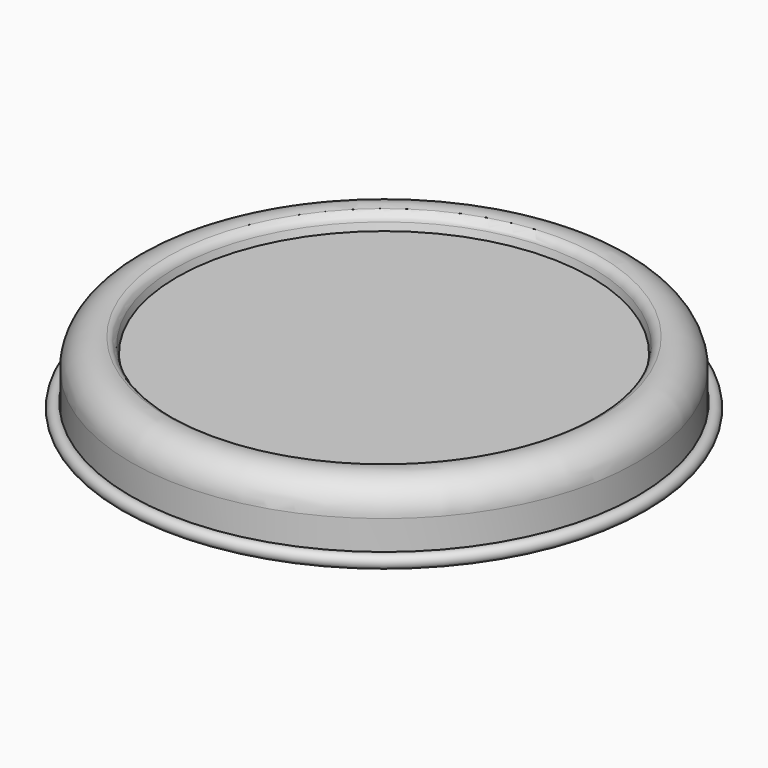
from build123d import *

# Parameters (mm, degrees)
F0_R     = 19.25
F1_DEPTH = 2.6185
F6_T     = 0.15


# Not quite as in the source:
# - a shell that OpenCascade refuses in one call is made with other operations: the cavity is built on its own and cut out


with BuildPart() as f1:
    # F0 (on Top) → F1 (new body)
    with BuildSketch(Plane.XY):
        Circle(F0_R)
    extrude(amount=F1_DEPTH)

    # F2 (on Front) → F3 (revolve)
    with BuildSketch(Plane.XZ):
        with BuildLine():
            Line((-19.39, 0.28), (-19.3, 0.4))
            ThreePointArc((-19.3, 0.4), (-20.0472135955, -0.2236067977), (-19.1, 0))
            Line((-19.1, 0), (-19.25, 0))
            ThreePointArc((-19.25, 0), (-19.9130495168, -0.1565247584), (-19.39, 0.28))
        make_face()
    revolve(axis=Axis((0, 0, 0), (0, 0, 1)))

    # F4 (on Front) → F5 (revolve)
    with BuildSketch(Plane.XZ):
        with BuildLine():
            ThreePointArc((-15.8901444738, 4.2056334644), (-16.1010152989, 4.5800338413), (-16.4751795318, 4.7913233913))
            ThreePointArc((-16.4751795318, 4.7913233913), (-18.3917322337, 4.3806570674), (-19.25, 2.6185))
            Line((-19.25, 2.6185), (-15.5, 2.6185))
            Line((-15.5, 2.6185), (0, 2.6185))
            Line((0, 2.6185), (0, 3.656625))
            Line((0, 3.656625), (-15.75518883, 3.656625))
            Line((-15.75518883, 3.656625), (-15.8901444738, 4.2056334644))
        make_face()
    revolve(axis=Axis((0, 0, 2.6185), (0, 0, 1)))

    # F6: shell of thickness 0.15, made by hand


with BuildPart() as f6_core1:
    # F6_t2: copy of F1
    add(f1.part)

    # the walls: a layer under each face that stays
    f6_faces = [f6_core1.faces().sort_by_distance(p)[0] for p in [
        (-19.25, 0, 1.30925),
        (18.3917322337, 0, 4.3806570674),
        (19.9130495168, 0, -0.1565247584),
        (16.1010152989, 0, 4.5800338413),
        (19.345, 0, 0.34),
        (15.8226666519, 0, 3.9311292322),
        (20.0472135955, 0, -0.2236067977),
        (0, 0, 3.656625),
    ]]
    thicken(f6_faces, amount=-F6_T, mode=Mode.SUBTRACT)

    # F6_s3 → F6_t4 (revolve, cut)
    with BuildSketch(Plane.XZ):
        Polygon((-15.7537321939, 3.658483066), (-15.9008524405, 3.6208184003), (-15.8727817552, 3.506625), (-15.75518883, 3.506625), align=None)
    revolve(axis=Axis((0, 0, 3.656625), (0, 0, 1)), mode=Mode.SUBTRACT)


with BuildPart() as f1_1:
    add(f1.part)

    # what is left inside the walls is the cavity
    f6_cavity = [f6_core1.part.solids().sort_by_distance(p)[0] for p in [
        (0, -6.366667, 0.0015),
    ]]
    add(f6_cavity, mode=Mode.SUBTRACT)


solid = f1_1.part
